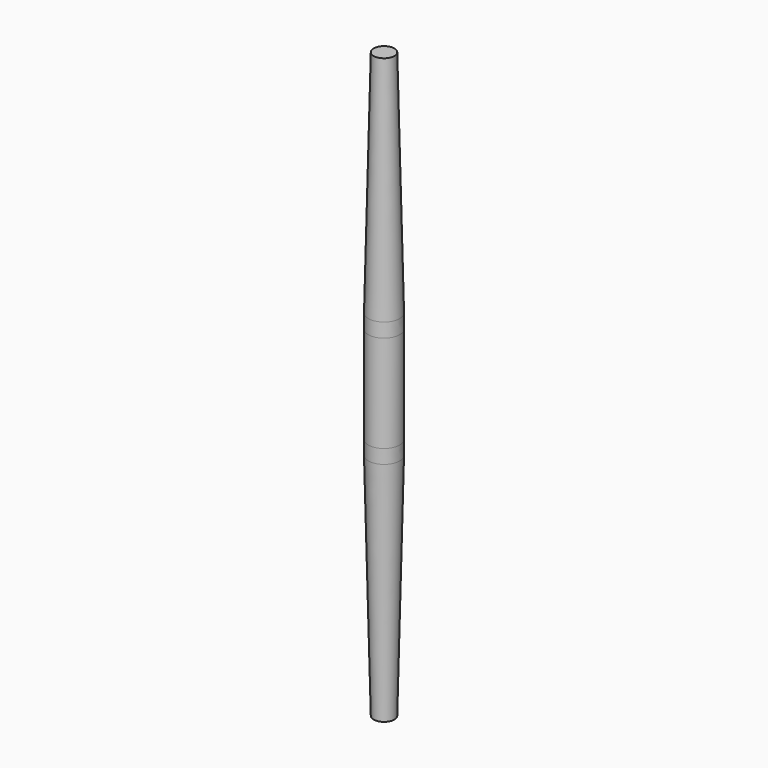
from build123d import *


# Not quite as in the source:
# - a feature names something its author has since deleted; it is built from what else it names


with BuildPart() as f1:
    # F0 (on Front) → F1 (revolve)
    with BuildSketch(Plane.XZ):
        with BuildLine():
            Line((0, 480), (0, 0))
            Line((0, 0), (0, -480))
            Line((0, -480), (17, -480))
            Line((17, -480), (25.7319285466, -102.9642244203))
            ThreePointArc((25.7319285466, -102.9642244203), (25.9329798908, -91.3883962972), (26, -79.8110163396))
            Line((26, -79.8110163396), (26, 0))
            Line((26, 0), (26, 79.8110163396))
            ThreePointArc((26, 79.8110163396), (25.9329798908, 91.3883962972), (25.7319285466, 102.9642244203))
            Line((25.7319285466, 102.9642244203), (17, 480))
            Line((17, 480), (0, 480))
        make_face()
    revolve(axis=Axis((0, 0, 240), (0, 0, 1)))


solid = f1.part
